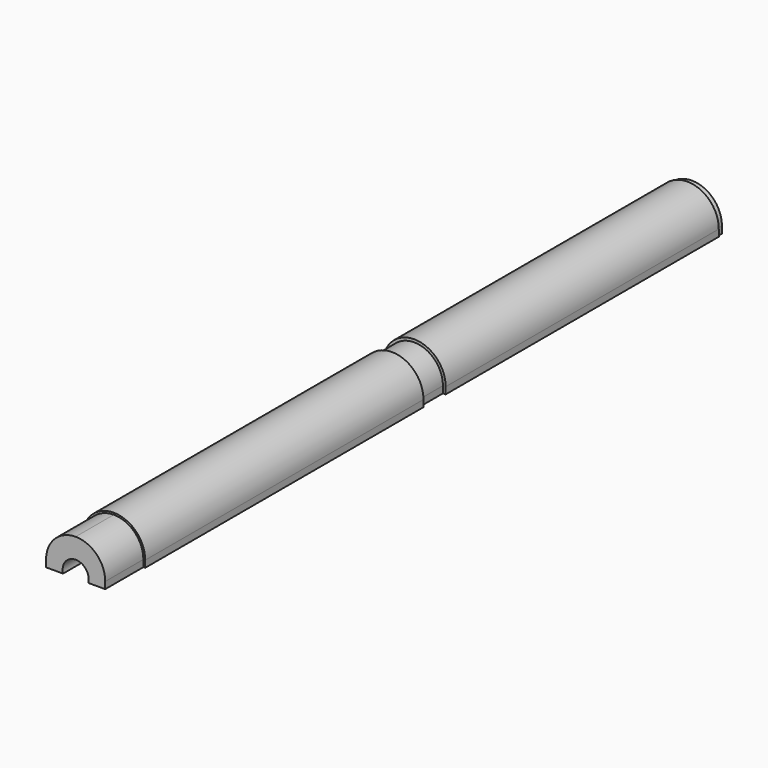
from build123d import *
from build123d import SkipClean  # not in build123d's __all__

# Parameters (mm, degrees)
F1_DEPTH  = 29.21
F3_DEPTH  = 160.5534
F5_DEPTH  = 15.4178
F7_DEPTH  = 42.5196
F9_DEPTH  = 177.3174
F11_DEPTH = 26.4922
F13_DEPTH = 3.1496


with BuildPart() as f1:
    # F0 (on Front) → F1 (new body)
    with BuildSketch(Plane.XZ):
        with BuildLine():
            Line((11.9332703397, -4.6441399077), (17.4498, -4.6441399077))
            Line((17.4498, -4.6441399077), (17.4498, -0.8595399077))
            ThreePointArc((17.4498, -0.8595399077), (0, 16.6918600923), (-17.4498, -0.8595399077))
            Line((-17.4498, -0.8595399077), (-17.4498, -4.6441399077))
            Line((-17.4498, -4.6441399077), (-11.9332703397, -4.6441399077))
            ThreePointArc((-11.9332703397, -4.6441399077), (0, 9.1988600923), (11.9332703397, -4.6441399077))
        make_face()
    extrude(amount=F1_DEPTH)

    # F2 (on face) → F3 (join)
    with BuildSketch(Plane.XZ.offset(29.21)):
        with BuildLine():
            ThreePointArc((-9.1113708093, -4.6441399077), (0, 6.4977884545), (9.1113708093, -4.6441399077))
            Line((9.1113708093, -4.6441399077), (11.9332703397, -4.6441399077))
            ThreePointArc((11.9332703397, -4.6441399077), (0, 9.1988600923), (-11.9332703397, -4.6441399077))
            Line((-11.9332703397, -4.6441399077), (-9.1113708093, -4.6441399077))
        make_face()
        with BuildLine():
            ThreePointArc((-11.9332703397, -4.6441399077), (0, 9.1988600923), (11.9332703397, -4.6441399077))
            Line((11.9332703397, -4.6441399077), (17.4498, -4.6441399077))
            Line((17.4498, -4.6441399077), (17.4498, -0.8595399077))
            ThreePointArc((17.4498, -0.8595399077), (0, 16.6918600923), (-17.4498, -0.8595399077))
            Line((-17.4498, -0.8595399077), (-17.4498, -4.6441399077))
            Line((-17.4498, -4.6441399077), (-11.9332703397, -4.6441399077))
        make_face()
    extrude(amount=F3_DEPTH)

    # F4 (on face) → F5 (join)
    with BuildSketch(Plane.XZ.offset(189.7634)):
        with BuildLine():
            Line((15.9258256822, -4.6441399077), (15.9258256822, -0.850692377))
            ThreePointArc((15.9258256822, -0.850692377), (0, 15.1678600923), (-15.9258256822, -0.850692377))
            Line((-15.9258256822, -0.850692377), (-15.9038025792, -4.6441399077))
            Line((-15.9038025792, -4.6441399077), (-9.1113708093, -4.6441399077))
            ThreePointArc((-9.1113708093, -4.6441399077), (0, 6.4977884545), (9.1113708093, -4.6441399077))
            Line((9.1113708093, -4.6441399077), (15.9258256822, -4.6441399077))
        make_face()
    extrude(amount=F5_DEPTH)

    # F6 (on face) → F7 (join)
    with BuildSketch(Plane.XZ.offset(205.1812)):
        with BuildLine():
            ThreePointArc((-9.1113708093, -4.6441399077), (0, 6.4977884545), (9.1113708093, -4.6441399077))
            Line((9.1113708093, -4.6441399077), (15.9258256822, -4.6441399077))
            Line((15.9258256822, -4.6441399077), (15.9258256822, -0.850692377))
            ThreePointArc((15.9258256822, -0.850692377), (0, 15.1678600923), (-15.9258256822, -0.850692377))
            Line((-15.9258256822, -0.850692377), (-15.9038025792, -4.6441399077))
            Line((-15.9038025792, -4.6441399077), (-9.1113708093, -4.6441399077))
        make_face()
        with BuildLine():
            Line((15.9258256822, -0.850692377), (15.9258256822, -4.6441399077))
            Line((15.9258256822, -4.6441399077), (17.4498, -4.6441399077))
            Line((17.4498, -4.6441399077), (17.4498, -0.8595399077))
            ThreePointArc((17.4498, -0.8595399077), (0, 16.6918600923), (-17.4498, -0.8595399077))
            Line((-17.4498, -0.8595399077), (-17.4498, -4.6441399077))
            Line((-17.4498, -4.6441399077), (-15.9038025792, -4.6441399077))
            Line((-15.9038025792, -4.6441399077), (-15.9258256822, -0.850692377))
            ThreePointArc((-15.9258256822, -0.850692377), (0, 15.1678600923), (15.9258256822, -0.850692377))
        make_face()
    extrude(amount=F7_DEPTH)

    # F8 (on face) → F9 (join)
    with BuildSketch(Plane.XZ.offset(247.7008)):
        with BuildLine():
            ThreePointArc((9.1113708093, -4.6441399077), (0, 6.4977884545), (-9.1113708093, -4.6441399077))
            Line((-9.1113708093, -4.6441399077), (-6.9997961445, -4.6441399077))
            ThreePointArc((-6.9997961445, -4.6441399077), (0, 4.4403884545), (6.9997961445, -4.6441399077))
            Line((6.9997961445, -4.6441399077), (9.1113708093, -4.6441399077))
        make_face()
        with BuildLine():
            ThreePointArc((17.4498, -0.8595399077), (0, 16.6918600923), (-17.4498, -0.8595399077))
            Line((-17.4498, -0.8595399077), (-17.4498, -4.6441399077))
            Line((-17.4498, -4.6441399077), (-9.1113708093, -4.6441399077))
            ThreePointArc((-9.1113708093, -4.6441399077), (0, 6.4977884545), (9.1113708093, -4.6441399077))
            Line((9.1113708093, -4.6441399077), (17.4498, -4.6441399077))
            Line((17.4498, -4.6441399077), (17.4498, -0.8595399077))
        make_face()
    extrude(amount=F9_DEPTH)

    # F10 (on face) → F11 (cut)
    with BuildSketch(Plane.XZ.offset(425.0182)):
        with BuildLine():
            ThreePointArc((0, 15.6758600923), (11.6553662483, 10.8276145233), (16.4338, -0.8565464805))
            Line((16.4338, -0.8565464805), (16.4338, -4.6441399077))
            Line((16.4338, -4.6441399077), (17.4498, -4.6441399077))
            Line((17.4498, -4.6441399077), (17.4498, -0.8595399077))
            ThreePointArc((17.4498, -0.8595399077), (0, 16.6918600923), (-17.4498, -0.8595399077))
            Line((-17.4498, -0.8595399077), (-17.4498, -4.6441399077))
            Line((-17.4498, -4.6441399077), (-16.4338, -4.6441399077))
            Line((-16.4338, -4.6441399077), (-16.4338, -0.8565464804))
            ThreePointArc((-16.4338, -0.8565464804), (-11.6553662483, 10.8276145233), (0, 15.6758600923))
        make_face()
    extrude(amount=-F11_DEPTH, mode=Mode.SUBTRACT)

    # F12 (on face) → F13 (join)
    with BuildSketch(Plane(origin=(0, 0, 0), x_dir=(-1, 0, 0), z_dir=(0, 1, 0))):
        with BuildLine():
            ThreePointArc((16.6878128411, -0.8551161423), (0, 15.9298600923), (-16.6878128411, -0.8551161423))
            Line((-16.6878128411, -0.8551161423), (-16.6878128411, -4.6441399077))
            Line((-16.6878128411, -4.6441399077), (-11.9332703397, -4.6441399077))
            ThreePointArc((-11.9332703397, -4.6441399077), (0, 9.1988600923), (11.9332703397, -4.6441399077))
            Line((11.9332703397, -4.6441399077), (16.6658154206, -4.6441399077))
            Line((16.6658154206, -4.6441399077), (16.6878128411, -0.8551161423))
        make_face()
    with SkipClean():  # cleaning this boolean's faces spoils the solid; the shape is the same uncleaned
        extrude(amount=F13_DEPTH)


solid = f1.part
